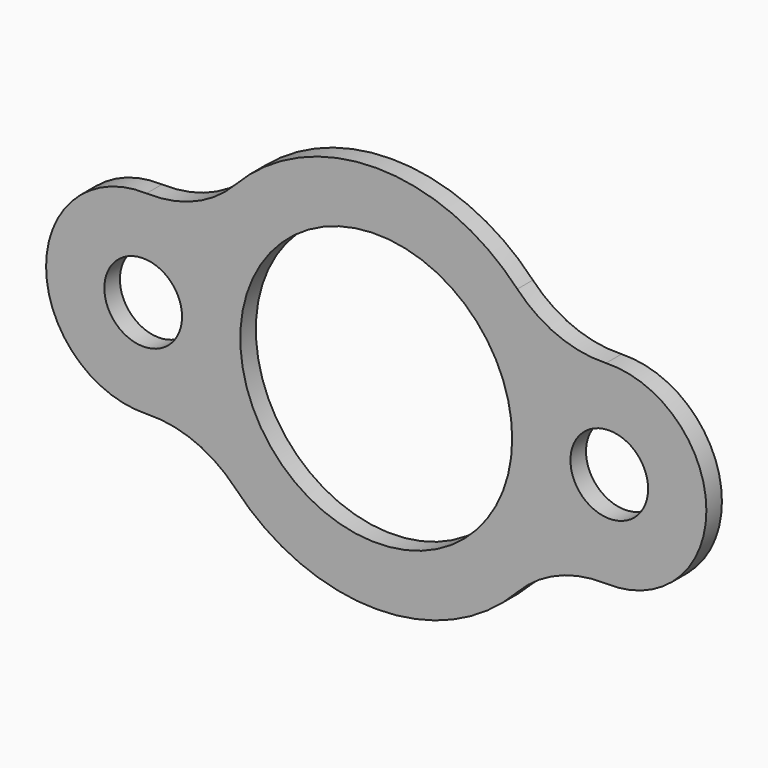
from build123d import *

# Parameters (mm, degrees)
F0_R     = 12.7
F0_R_2   = 44.45
F1_DEPTH = 6.35


# Not quite as in the source:
# - a length typed as a fraction of an inch, garbled in the dataset ("3 / 203.2 mm" for 3/8 in), is restored


with BuildPart() as f1:
    # F0 (on Front) → F1 (new body)
    with BuildSketch(Plane.XZ):
        with BuildLine():
            ThreePointArc((-75.1176136364, -31.7315448688), (-59.3475236203, -34.5646316236), (-46.13671875, -43.6308741946))
            ThreePointArc((-46.13671875, -43.6308741946), (0, -63.5), (46.13671875, -43.6308741946))
            ThreePointArc((46.13671875, -43.6308741946), (59.3475236203, -34.5646316236), (75.1176136364, -31.7315448688))
            ThreePointArc((75.1176136364, -31.7315448688), (107.95, 0), (75.1176136364, 31.7315448688))
            ThreePointArc((75.1176136364, 31.7315448688), (59.3475236203, 34.5646316236), (46.13671875, 43.6308741946))
            ThreePointArc((46.13671875, 43.6308741946), (0, 63.5), (-46.13671875, 43.6308741946))
            ThreePointArc((-46.13671875, 43.6308741946), (-59.3475236203, 34.5646316236), (-75.1176136364, 31.7315448688))
            ThreePointArc((-75.1176136364, 31.7315448688), (-107.95, 0), (-75.1176136364, -31.7315448688))
        make_face()
        with Locations((-76.2, 0)):
            Circle(F0_R, mode=Mode.SUBTRACT)
        Circle(F0_R_2, mode=Mode.SUBTRACT)
        with Locations((76.2, 0)):
            Circle(F0_R, mode=Mode.SUBTRACT)
    extrude(amount=F1_DEPTH)


solid = f1.part
